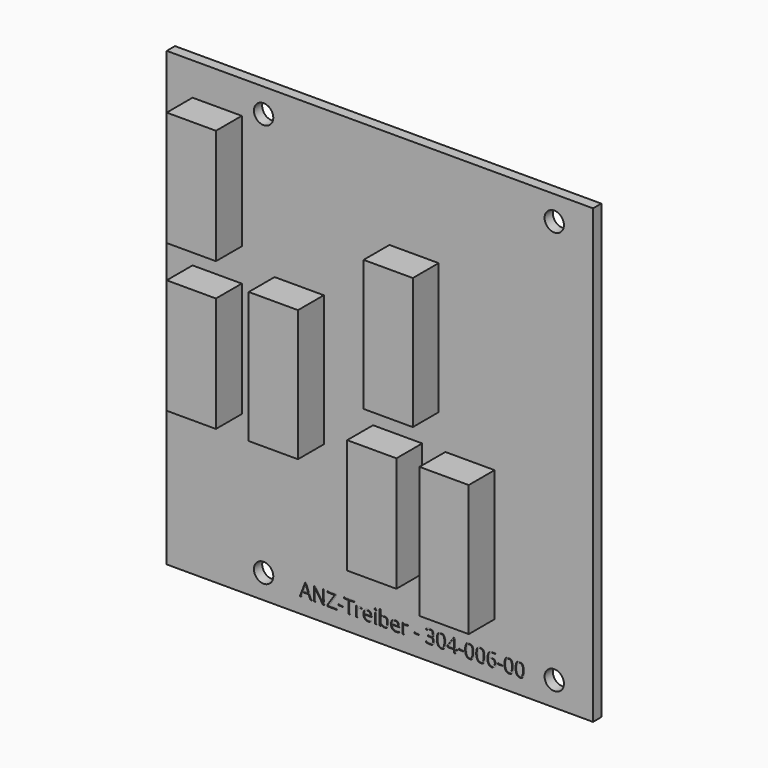
from build123d import *

# Parameters (mm, degrees)
F0_W         = 66
F0_H         = 70
F0_R         = 1.5
F0_W_2       = 7.62
F0_H_2       = 17.78
F0_H_3       = 20.32
F1_DEPTH     = 1.6
F2_TEXT_SIZE = 2.988698982
F3_DEPTH     = 0.1
F4_DEPTH     = 5


# Not quite as in the source:
# - Text() gives the source's letters only with a copy of the font that has no kerning and outlines rounded to 1/6400 em; it was checked with that copy


with BuildPart() as f1:
    # F0 (on Front) → F1 (new body)
    with BuildSketch(Plane.XZ):
        Rectangle(F0_W, F0_H)
        with Locations((-18, -31.25)):
            Circle(F0_R, mode=Mode.SUBTRACT)
        with Locations((-25.19, -1.83)):
            Rectangle(F0_W_2, F0_H_2, mode=Mode.SUBTRACT)
        with Locations((-12.49, -0.56)):
            Rectangle(F0_W_2, F0_H_3, mode=Mode.SUBTRACT)
        with Locations((27, -31.25)):
            Circle(F0_R, mode=Mode.SUBTRACT)
        with Locations((2.75, -14.53)):
            Rectangle(F0_W_2, F0_H_2, mode=Mode.SUBTRACT)
        with Locations((13.95, -15.8)):
            Rectangle(F0_W_2, F0_H_3, mode=Mode.SUBTRACT)
        with Locations((-25.19, 21.03)):
            Rectangle(F0_W_2, F0_H_2, mode=Mode.SUBTRACT)
        with Locations((-18, 31.25)):
            Circle(F0_R, mode=Mode.SUBTRACT)
        with Locations((5.29, 9.6)):
            Rectangle(F0_W_2, F0_H_3, mode=Mode.SUBTRACT)
        with Locations((27, 31.25)):
            Circle(F0_R, mode=Mode.SUBTRACT)
        with Locations((-25.19, 21.03)):
            Rectangle(F0_W_2, F0_H_2)
        with Locations((-25.19, -1.83)):
            Rectangle(F0_W_2, F0_H_2)
        with Locations((-12.49, -0.56)):
            Rectangle(F0_W_2, F0_H_3)
        with Locations((5.29, 9.6)):
            Rectangle(F0_W_2, F0_H_3)
        with Locations((2.75, -14.53)):
            Rectangle(F0_W_2, F0_H_2)
        with Locations((13.95, -15.8)):
            Rectangle(F0_W_2, F0_H_3)
    extrude(amount=-F1_DEPTH)

    # F2 (on face) → F3 (cut)
    with BuildSketch(Plane.XZ):
        with Locations((-12.3948364708, -32.6221378567)):
            Text('ANZ-Treiber - 304-006-00', F2_TEXT_SIZE, font='Open Sans', text_align=(TextAlign.LEFT, TextAlign.BOTTOM))
    extrude(amount=-F3_DEPTH, mode=Mode.SUBTRACT)

    # F0 (on Front) → F4 (join)
    with BuildSketch(Plane.XZ):
        with Locations((-25.19, 21.03)):
            Rectangle(F0_W_2, F0_H_2)
        with Locations((-25.19, -1.83)):
            Rectangle(F0_W_2, F0_H_2)
        with Locations((-12.49, -0.56)):
            Rectangle(F0_W_2, F0_H_3)
        with Locations((5.29, 9.6)):
            Rectangle(F0_W_2, F0_H_3)
        with Locations((2.75, -14.53)):
            Rectangle(F0_W_2, F0_H_2)
        with Locations((13.95, -15.8)):
            Rectangle(F0_W_2, F0_H_3)
    extrude(amount=F4_DEPTH)


solid = f1.part
